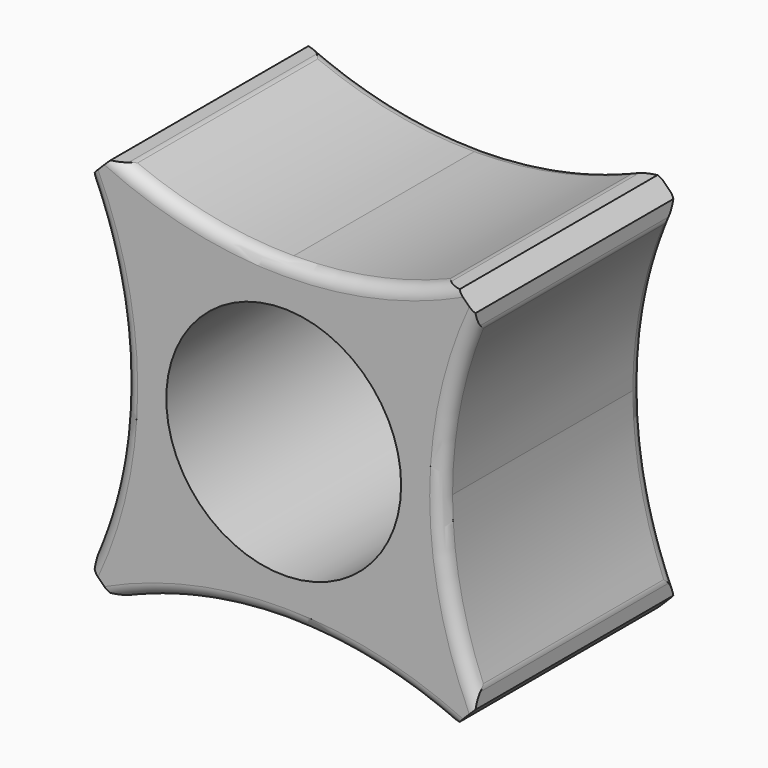
from build123d import *

# Parameters (mm, degrees)
F1_DEPTH     = 10.033
F2_T1_DEPTH  = 10.536999752
F2_T4_ANGLE  = 54.0553597126
F2_T6_ANGLE  = 54.0553597126
F2_T8_ANGLE  = 54.0553597126
F2_T10_ANGLE = 54.0553597126
F2_T12_ANGLE = 54.0553597126
F2_T14_ANGLE = 54.0553597126
F2_T16_ANGLE = 54.0553597126
F2_T18_ANGLE = 54.0553597126


# Not quite as in the source:
# - a fillet or chamfer that OpenCascade refuses, or shapes differently, is made with other operations: its cross-section is extruded or revolved along the edge and cut away or added


with BuildPart() as f1:
    # F0 (on Front) → F1 (new body)
    with BuildSketch(Plane.XZ):
        with BuildLine():
            ThreePointArc((-4.699, 0), (0, 4.699), (4.699, 0))
            Line((4.699, 0), (6.35, 0))
            ThreePointArc((6.35, 0), (6.6706130443, 3.2378773911), (7.62, 6.35))
            Line((7.62, 6.35), (7.62, 6.985))
            Line((7.62, 6.985), (6.985, 7.62))
            Line((6.985, 7.62), (6.35, 7.62))
            ThreePointArc((6.35, 7.62), (3.2378773911, 6.6706130443), (0, 6.35))
            ThreePointArc((0, 6.35), (-3.2378773911, 6.6706130443), (-6.35, 7.62))
            Line((-6.35, 7.62), (-6.985, 7.62))
            Line((-6.985, 7.62), (-7.62, 6.985))
            Line((-7.62, 6.985), (-7.62, 6.35))
            ThreePointArc((-7.62, 6.35), (-6.6706130443, 3.2378773911), (-6.35, 0))
            Line((-6.35, 0), (-4.699, 0))
        make_face()
        with BuildLine():
            Line((6.35, 0), (4.699, 0))
            ThreePointArc((4.699, 0), (0, -4.699), (-4.699, 0))
            Line((-4.699, 0), (-6.35, 0))
            ThreePointArc((-6.35, 0), (-6.6706130443, -3.2378773911), (-7.62, -6.35))
            Line((-7.62, -6.35), (-7.62, -6.985))
            Line((-7.62, -6.985), (-6.985, -7.62))
            Line((-6.985, -7.62), (-6.35, -7.62))
            ThreePointArc((-6.35, -7.62), (-3.2378773911, -6.6706130443), (0, -6.35))
            ThreePointArc((0, -6.35), (3.2378773911, -6.6706130443), (6.35, -7.62))
            Line((6.35, -7.62), (6.985, -7.62))
            Line((6.985, -7.62), (7.62, -6.985))
            Line((7.62, -6.985), (7.62, -6.35))
            ThreePointArc((7.62, -6.35), (6.6706130443, -3.2378773911), (6.35, 0))
        make_face()
    extrude(amount=F1_DEPTH)

    # F2: fillet of radius 0.508 on 16 edges, made by hand

    # F2_s2 → F2_t1 (cut)
    with BuildSketch(Plane.XZ.offset(-0.251999876)):
        with BuildLine():
            ThreePointArc((-7.5820895522, 6.2582387578), (-7.6104322885, 6.3526711894), (-7.62, 6.4507999504))
            Line((-7.62, 6.4507999504), (-7.62, 6.35))
            ThreePointArc((-7.62, 6.35), (-7.6009757994, 6.3041478761), (-7.5820895522, 6.2582387578))
        make_face()
        with BuildLine():
            ThreePointArc((-7.5820895522, -6.2582387578), (-7.6104322885, -6.3526711894), (-7.62, -6.4507999504))
            Line((-7.62, -6.4507999504), (-7.62, -6.35))
            ThreePointArc((-7.62, -6.35), (-7.6009757994, -6.3041478761), (-7.5820895522, -6.2582387578))
        make_face()
        with BuildLine():
            ThreePointArc((6.4507999504, 7.62), (6.3526711894, 7.6104322885), (6.2582387578, 7.5820895522))
            ThreePointArc((6.2582387578, 7.5820895522), (6.3041478761, 7.6009757994), (6.35, 7.62))
            Line((6.35, 7.62), (6.4507999504, 7.62))
        make_face()
        with BuildLine():
            ThreePointArc((-6.2582387578, 7.5820895522), (-6.3526711894, 7.6104322885), (-6.4507999504, 7.62))
            Line((-6.4507999504, 7.62), (-6.35, 7.62))
            ThreePointArc((-6.35, 7.62), (-6.3041478761, 7.6009757994), (-6.2582387578, 7.5820895522))
        make_face()
        with BuildLine():
            ThreePointArc((7.62, -6.4507999504), (7.6104322885, -6.3526711894), (7.5820895522, -6.2582387578))
            ThreePointArc((7.5820895522, -6.2582387578), (7.6009757994, -6.3041478761), (7.62, -6.35))
            Line((7.62, -6.35), (7.62, -6.4507999504))
        make_face()
        with BuildLine():
            ThreePointArc((7.5820895522, 6.2582387578), (7.6104322885, 6.3526711894), (7.62, 6.4507999504))
            Line((7.62, 6.4507999504), (7.62, 6.35))
            ThreePointArc((7.62, 6.35), (7.6009757994, 6.3041478761), (7.5820895522, 6.2582387578))
        make_face()
        with BuildLine():
            ThreePointArc((-6.4507999504, -7.62), (-6.3526711894, -7.6104322885), (-6.2582387578, -7.5820895522))
            ThreePointArc((-6.2582387578, -7.5820895522), (-6.3041478761, -7.6009757994), (-6.35, -7.62))
            Line((-6.35, -7.62), (-6.4507999504, -7.62))
        make_face()
        with BuildLine():
            ThreePointArc((6.2582387578, -7.5820895522), (6.3526711894, -7.6104322885), (6.4507999504, -7.62))
            Line((6.4507999504, -7.62), (6.35, -7.62))
            ThreePointArc((6.35, -7.62), (6.3041478761, -7.6009757994), (6.2582387578, -7.5820895522))
        make_face()
    extrude(amount=F2_T1_DEPTH, mode=Mode.SUBTRACT)

    # F2_s3 → F2_t4 (revolve, cut)
    with BuildSketch(Plane(origin=(-4.7205523, 0, 9.2535512946), x_dir=(0, 1, 0), z_dir=(-0.4544208961, 0, 0.8907870953))):
        with BuildLine():
            ThreePointArc((-0.508, 3.8533929988), (-0.1487897552, 3.7046032436), (0, 3.3453929988))
            Line((0, 3.3453929988), (0, 3.8533929988))
            Line((0, 3.8533929988), (-0.508, 3.8533929988))
        make_face()
    revolve(axis=Axis((-22.86, 0, 0), (0, 1, 0)), revolution_arc=F2_T4_ANGLE, mode=Mode.SUBTRACT)

    # F2_s5 → F2_t6 (revolve, cut)
    with BuildSketch(Plane(origin=(-4.7205523, 0, 9.2535512946), x_dir=(0, 1, 0), z_dir=(-0.4544208961, 0, 0.8907870953))):
        with BuildLine():
            ThreePointArc((-9.525, 3.8533929988), (-9.8842102448, 3.7046032436), (-10.033, 3.3453929988))
            Line((-10.033, 3.3453929988), (-10.033, 3.8533929988))
            Line((-10.033, 3.8533929988), (-9.525, 3.8533929988))
        make_face()
    revolve(axis=Axis((-22.86, -10.033, 0), (0, 1, 0)), revolution_arc=F2_T6_ANGLE, mode=Mode.SUBTRACT)

    # F2_s7 → F2_t8 (revolve, cut)
    with BuildSketch(Plane(origin=(9.2535512946, 0, 4.7205523), x_dir=(0, 1, 0), z_dir=(0.8907870953, 0, 0.4544208961))):
        with BuildLine():
            ThreePointArc((-0.508, 3.8533929988), (-0.1487897552, 3.7046032436), (0, 3.3453929988))
            Line((0, 3.3453929988), (0, 3.8533929988))
            Line((0, 3.8533929988), (-0.508, 3.8533929988))
        make_face()
    revolve(axis=Axis((0, 0, 22.86), (0, 1, 0)), revolution_arc=F2_T8_ANGLE, mode=Mode.SUBTRACT)

    # F2_s9 → F2_t10 (revolve, cut)
    with BuildSketch(Plane(origin=(9.2535512946, 0, 4.7205523), x_dir=(0, 1, 0), z_dir=(0.8907870953, 0, 0.4544208961))):
        with BuildLine():
            ThreePointArc((-9.525, 3.8533929988), (-9.8842102448, 3.7046032436), (-10.033, 3.3453929988))
            Line((-10.033, 3.3453929988), (-10.033, 3.8533929988))
            Line((-10.033, 3.8533929988), (-9.525, 3.8533929988))
        make_face()
    revolve(axis=Axis((0, -10.033, 22.86), (0, 1, 0)), revolution_arc=F2_T10_ANGLE, mode=Mode.SUBTRACT)

    # F2_s11 → F2_t12 (revolve, cut)
    with BuildSketch(Plane(origin=(4.7205523, 0, -9.2535512946), x_dir=(0, 1, 0), z_dir=(0.4544208961, 0, -0.8907870953))):
        with BuildLine():
            ThreePointArc((-0.508, 3.8533929988), (-0.1487897552, 3.7046032436), (0, 3.3453929988))
            Line((0, 3.3453929988), (0, 3.8533929988))
            Line((0, 3.8533929988), (-0.508, 3.8533929988))
        make_face()
    revolve(axis=Axis((22.86, 0, 0), (0, 1, 0)), revolution_arc=F2_T12_ANGLE, mode=Mode.SUBTRACT)

    # F2_s13 → F2_t14 (revolve, cut)
    with BuildSketch(Plane(origin=(4.7205523, 0, -9.2535512946), x_dir=(0, 1, 0), z_dir=(0.4544208961, 0, -0.8907870953))):
        with BuildLine():
            ThreePointArc((-9.525, 3.8533929988), (-9.8842102448, 3.7046032436), (-10.033, 3.3453929988))
            Line((-10.033, 3.3453929988), (-10.033, 3.8533929988))
            Line((-10.033, 3.8533929988), (-9.525, 3.8533929988))
        make_face()
    revolve(axis=Axis((22.86, -10.033, 0), (0, 1, 0)), revolution_arc=F2_T14_ANGLE, mode=Mode.SUBTRACT)

    # F2_s15 → F2_t16 (revolve, cut)
    with BuildSketch(Plane(origin=(-9.2535512946, 0, -4.7205523), x_dir=(0, 1, 0), z_dir=(-0.8907870953, 0, -0.4544208961))):
        with BuildLine():
            ThreePointArc((-0.508, 3.8533929988), (-0.1487897552, 3.7046032436), (0, 3.3453929988))
            Line((0, 3.3453929988), (0, 3.8533929988))
            Line((0, 3.8533929988), (-0.508, 3.8533929988))
        make_face()
    revolve(axis=Axis((0, 0, -22.86), (0, 1, 0)), revolution_arc=F2_T16_ANGLE, mode=Mode.SUBTRACT)

    # F2_s17 → F2_t18 (revolve, cut)
    with BuildSketch(Plane(origin=(-9.2535512946, 0, -4.7205523), x_dir=(0, 1, 0), z_dir=(-0.8907870953, 0, -0.4544208961))):
        with BuildLine():
            ThreePointArc((-9.525, 3.8533929988), (-9.8842102448, 3.7046032436), (-10.033, 3.3453929988))
            Line((-10.033, 3.3453929988), (-10.033, 3.8533929988))
            Line((-10.033, 3.8533929988), (-9.525, 3.8533929988))
        make_face()
    revolve(axis=Axis((0, -10.033, -22.86), (0, 1, 0)), revolution_arc=F2_T18_ANGLE, mode=Mode.SUBTRACT)


solid = f1.part
